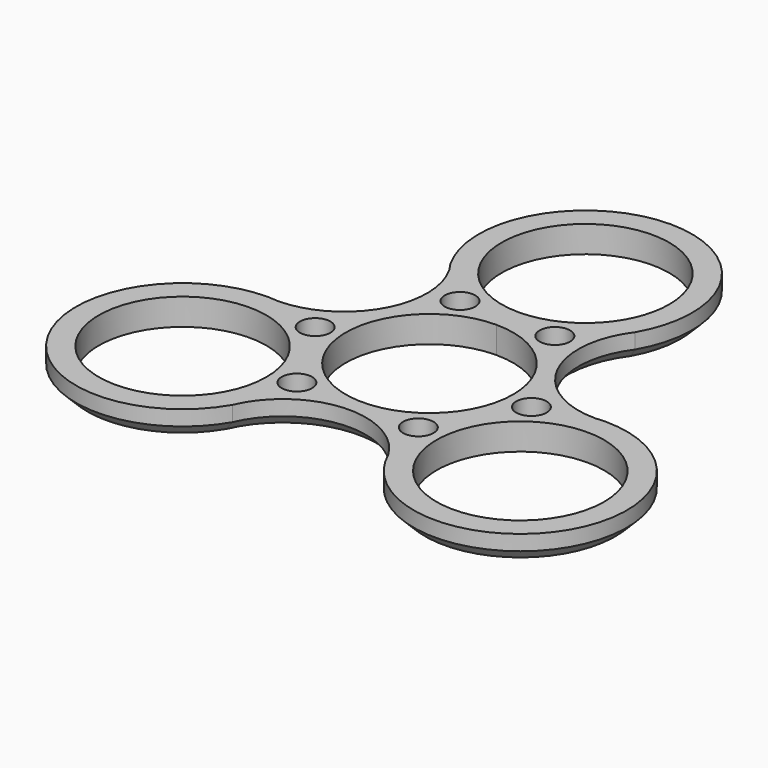
from build123d import *

# Parameters (mm, degrees)
F0_R       = 11
F0_R_2     = 2
F1_DEPTH   = 3.5
F2_C1_SIZE = 1.5
F2_C2_SIZE = 1.5
F2_C3_SIZE = 1.5
F2_C4_SIZE = 1.5
F2_C5_SIZE = 1.5
F2_C6_SIZE = 1.5


with BuildPart() as f1:
    # F0 (on Top) → F1 (new body)
    with BuildSketch(Plane.XY):
        with BuildLine():
            ThreePointArc((22.164837833, 1.2031249106), (11.390396953, 6.576248747), (12.124355653, 18.5937501788))
            ThreePointArc((12.124355653, 18.5937501788), (0, 39.5937501788), (-12.124355653, 18.5937501788))
            ThreePointArc((-12.124355653, 18.5937501788), (-11.390396953, 6.576248747), (-22.164837833, 1.2031249106))
            ThreePointArc((-22.164837833, 1.2031249106), (-34.2891934859, -19.7968750894), (-10.04048218, -19.7968750894))
            ThreePointArc((-10.04048218, -19.7968750894), (0, -13.152497494), (10.04048218, -19.7968750894))
            ThreePointArc((10.04048218, -19.7968750894), (34.2891934859, -19.7968750894), (22.164837833, 1.2031249106))
        make_face()
        with Locations((-22.164837833, -12.7968750894)):
            Circle(F0_R, mode=Mode.SUBTRACT)
        with Locations((-7.9711980778, -11.7872301109)):
            Circle(F0_R_2, mode=Mode.SUBTRACT)
        with Locations((-14.1936397552, -1.0096449785)):
            Circle(F0_R_2, mode=Mode.SUBTRACT)
        with Locations((7.9711980778, -11.7872301109)):
            Circle(F0_R_2, mode=Mode.SUBTRACT)
        with Locations((22.164837833, -12.7968750894)):
            Circle(F0_R, mode=Mode.SUBTRACT)
        with BuildLine():
            ThreePointArc((0, 11), (7.7781745931, 7.7781745931), (11, 0))
            ThreePointArc((11, 0), (-7.7781745931, -7.7781745931), (0, 11))
        make_face(mode=Mode.SUBTRACT)
        with Locations((14.1936397552, -1.0096449785)):
            Circle(F0_R_2, mode=Mode.SUBTRACT)
        with Locations((-6.2224416774, 12.7968750894)):
            Circle(F0_R_2, mode=Mode.SUBTRACT)
        with Locations((6.2224416774, 12.7968750894)):
            Circle(F0_R_2, mode=Mode.SUBTRACT)
        with BuildLine():
            ThreePointArc((9.5262794416, 20.0937501788), (5.5, 16.0674707372), (0, 14.5937501788))
            ThreePointArc((0, 14.5937501788), (-5.5, 16.0674707372), (-9.5262794416, 20.0937501788))
            ThreePointArc((-9.5262794416, 20.0937501788), (-2.8470094961, 36.218934268), (11, 25.5937501788))
            ThreePointArc((11, 25.5937501788), (10.6251840892, 22.7467406827), (9.5262794416, 20.0937501788))
        make_face(mode=Mode.SUBTRACT)
    extrude(amount=F1_DEPTH)

    # F2: chamfer of 1.5 on 6 edges, made by hand

    # F2_c1
    f2_c1_edges = [f1.edges().sort_by_distance(p)[0] for p in [
        (0, -13.152497494, 0),
    ]]
    chamfer(f2_c1_edges, length=F2_C1_SIZE)

    # F2_c2
    f2_c2_edges = [f1.edges().sort_by_distance(p)[0] for p in [
        (-11.390396953, 6.576248747, 0),
    ]]
    chamfer(f2_c2_edges, length=F2_C2_SIZE)

    # F2_c3
    f2_c3_edges = [f1.edges().sort_by_distance(p)[0] for p in [
        (11.390396953, 6.576248747, 0),
    ]]
    chamfer(f2_c3_edges, length=F2_C3_SIZE)

    # F2_c4
    f2_c4_edges = [f1.edges().sort_by_distance(p)[0] for p in [
        (34.2891934859, -19.7968750894, 0),
    ]]
    chamfer(f2_c4_edges, length=F2_C4_SIZE)

    # F2_c5
    f2_c5_edges = [f1.edges().sort_by_distance(p)[0] for p in [
        (-34.2891934859, -19.7968750894, 0),
    ]]
    chamfer(f2_c5_edges, length=F2_C5_SIZE)

    # F2_c6
    f2_c6_edges = [f1.edges().sort_by_distance(p)[0] for p in [
        (0, 39.5937501788, 0),
    ]]
    chamfer(f2_c6_edges, length=F2_C6_SIZE)


solid = f1.part
